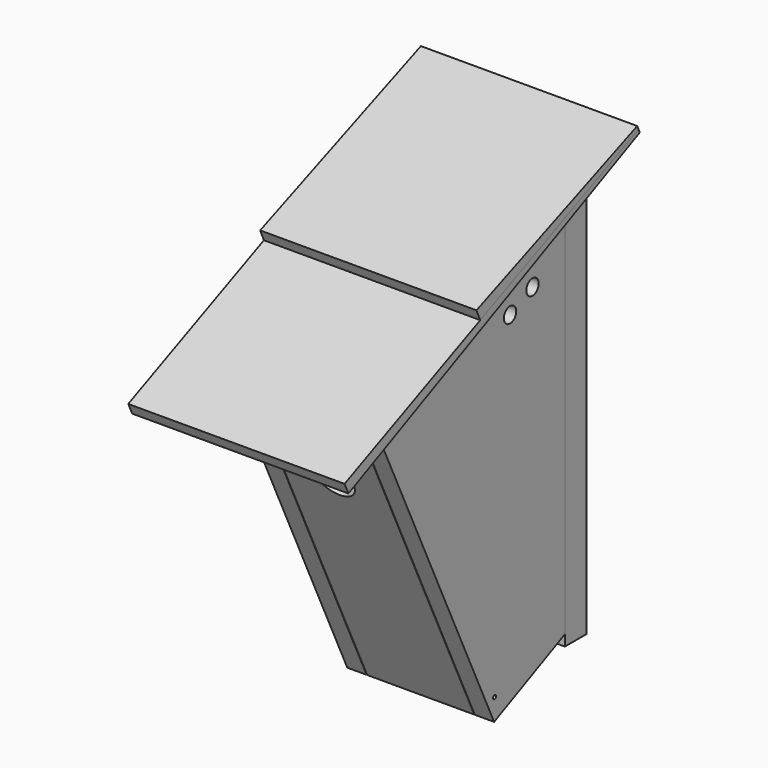
from build123d import *

# Parameters (mm, degrees)
F1_DEPTH       = 355.6
F3_DEPTH       = 60.326
F3_DEPTH_BACK  = 60.326
F5_DEPTH       = 44.45
F7_DEPTH       = 44.45
F8_R           = 1.5875
F8_R_2         = 6.35
F9_DEPTH       = 15.875
F10_R          = 1.5875
F10_R_2        = 6.35
F11_DEPTH      = 15.875
F13_DEPTH      = 15.875
F14_R          = 1.5875
F15_DEPTH      = 25.4
F16_R          = 1.5875
F17_DEPTH      = 25.4
F19_DEPTH      = 88.9
F21_DEPTH      = 88.9
F21_DEPTH_BACK = 88.9
F23_DEPTH      = 60.325
F24_R          = 1.3462
F25_DEPTH      = 38.1
F26_R          = 2.6924
F27_DEPTH      = 0.762
F29_R          = 1.5875
F31_R          = 0.762


with BuildPart() as f1:
    # F0 (on Top) → F1 (new body)
    with BuildSketch(Plane.XY):
        Polygon((60.325, 0), (-60.325, 0), (-60.325, -22.225), (-44.45, -22.225), (-44.45, -38.1), (44.45, -38.1), (44.45, -22.225), (60.325, -22.225), align=None)
    extrude(amount=-F1_DEPTH)

    # F2 (on Right) → F3 (cut, two sides)
    with BuildSketch(Plane.YZ) as f3_sk:
        Polygon((-38.1, -17.7663217757), (0, 0), (-38.1, 0), align=None)
    extrude(amount=-F3_DEPTH, mode=Mode.SUBTRACT)
    extrude(f3_sk.sketch, amount=F3_DEPTH_BACK, mode=Mode.SUBTRACT)


with BuildPart() as f5:
    # F4 (on Right) → F5 (new body, symmetric)
    with BuildSketch(Plane.YZ):
        Polygon((-38.1, -59.8050204882), (-38.1, -17.7663217757), (-209.3013597097, -97.5988268949), (-193.1996039373, -132.129153581), align=None)
    extrude(amount=F5_DEPTH, both=True)


with BuildPart() as f7:
    # F6 (on Right) → F7 (new body, symmetric)
    with BuildSketch(Plane.YZ):
        Polygon((-38.1, -326.5050204882), (-38.1, -284.4663217757), (-107.1493332197, -316.6645546466), (-91.0475774474, -351.1948813327), align=None)
    extrude(amount=F7_DEPTH, both=True)


with BuildPart() as f9:
    # F8 (on face) → F9 (new body, through all)
    with BuildSketch(Plane(origin=(-44.45, 0, 0), x_dir=(0, -1, 0), z_dir=(-1, 0, 0))):
        Polygon((223.6889958289, -104.3078918), (22.225, -10.3636877025), (22.225, -346.6732774023), (94.8749496503, -380.5505052888), align=None)
        with Locations((94.3901964958, -362.808336717)):
            Circle(F8_R, mode=Mode.SUBTRACT)
        with Locations((55.4660997165, -81.9158653491)):
            Circle(F8_R_2, mode=Mode.SUBTRACT)
        with Locations((78.4863175073, -92.6503691973)):
            Circle(F8_R_2, mode=Mode.SUBTRACT)
    extrude(amount=F9_DEPTH)


with BuildPart() as f11:
    # F10 (on face) → F11 (new body, through all)
    with BuildSketch(Plane.YZ.offset(44.45)):
        Polygon((-22.225, -346.6732774023), (-22.225, -10.3636877025), (-223.6889958289, -104.3078918), (-94.8749496503, -380.5505052888), align=None)
        with Locations((-94.3901964958, -362.808336717)):
            Circle(F10_R, mode=Mode.SUBTRACT)
        with Locations((-78.4863175073, -92.6503691973)):
            Circle(F10_R_2, mode=Mode.SUBTRACT)
        with Locations((-55.4660997165, -81.9158653491)):
            Circle(F10_R_2, mode=Mode.SUBTRACT)
    extrude(amount=F11_DEPTH)


with BuildPart() as f13:
    # F12 (on face) → F13 (new body)
    with BuildSketch(Plane(origin=(0, -223.6889958289, -104.3078918), x_dir=(1, 0, 0), z_dir=(0, -0.906307787, -0.4226182617))):
        with BuildLine():
            Line((-2.38125, -6.35), (-44.0436, -6.35))
            Line((-44.0436, -6.35), (-44.0436, -304.8))
            Line((-44.0436, -304.8), (44.0436, -304.8))
            Line((44.0436, -304.8), (44.0436, -6.35))
            Line((44.0436, -6.35), (2.38125, -6.35))
            Line((2.38125, -6.35), (2.38125, -12.7))
            ThreePointArc((2.38125, -12.7), (0, -15.08125), (-2.38125, -12.7))
            Line((-2.38125, -12.7), (-2.38125, -6.35))
        make_face()
        with BuildLine():
            ThreePointArc((17.4625, -90.4875), (0, -107.95), (-17.4625, -90.4875))
            Line((-17.4625, -90.4875), (-17.4625, -68.2625))
            ThreePointArc((-17.4625, -68.2625), (0, -50.8), (17.4625, -68.2625))
            Line((17.4625, -68.2625), (17.4625, -90.4875))
        make_face(mode=Mode.SUBTRACT)
    extrude(amount=-F13_DEPTH)

    # F14 (on face) → F15 (cut)
    with BuildSketch(Plane(origin=(-44.0436, 0, 0), x_dir=(0, -1, 0), z_dir=(-1, 0, 0))):
        with Locations((94.3901964958, -362.808336717)):
            Circle(F14_R)
    extrude(amount=-F15_DEPTH, mode=Mode.SUBTRACT)

    # F16 (on face) → F17 (cut)
    with BuildSketch(Plane.YZ.offset(44.0436)):
        with Locations((-94.3901964958, -362.808336717)):
            Circle(F16_R)
    extrude(amount=-F17_DEPTH, mode=Mode.SUBTRACT)


with BuildPart() as f19:
    # F18 (on Right) → F19 (new body, symmetric)
    with BuildSketch(Plane.YZ):
        Polygon((-284.2382702226, -122.0328074674), (-280.2128312795, -130.6653891389), (19.05, 8.8831608879), (17.708187019, 11.7606881117), align=None)
    extrude(amount=F19_DEPTH, both=True)


with BuildPart() as f21:
    # F20 (on Right) → F21 (new body, two sides)
    with BuildSketch(Plane.YZ) as f21_sk:
        Polygon((-144.8483111348, -60.2686455516), (17.708187019, 11.7606881117), (16.4219489178, 14.6634827216), (-148.7070254382, -51.5602617219), align=None)
    extrude(amount=F21_DEPTH)
    extrude(f21_sk.sketch, amount=-F21_DEPTH_BACK)


with BuildPart() as f23:
    # F22 (on Right) → F23 (new body, symmetric)
    with BuildSketch(Plane.YZ):
        Polygon((19.05, 8.8831608879), (0, 0), (0, -16.5168391121), (19.05, -16.5168391121), align=None)
    extrude(amount=F23_DEPTH, both=True)


with BuildPart() as f25:
    # F24 (on face) → F25 (new body)
    with BuildSketch(Plane(origin=(-60.325, 0, 0), x_dir=(0, -1, 0), z_dir=(-1, 0, 0))):
        with Locations((94.3901964958, -362.808336717)):
            Circle(F24_R)
    extrude(amount=-F25_DEPTH)

    # F26 (on face) → F27 (join)
    with BuildSketch(Plane(origin=(-60.325, 0, 0), x_dir=(0, -1, 0), z_dir=(-1, 0, 0))):
        with Locations((94.3901964958, -362.808336717)):
            Circle(F26_R)
    extrude(amount=F27_DEPTH)


with BuildPart() as f30:
    # F30: sweep along a path in F28
    with BuildLine(Plane.YZ) as f30_path:
        Line((-204.6050142761, -107.6701721783), (-216.1151231714, -113.0374241024))
        ThreePointArc((-216.1151231714, -113.0374241024), (-218.5776898064, -115.7248440056), (-218.4186945357, -119.3664344097))
        Line((-218.4186945357, -119.3664344097), (-216.4059750641, -123.6827252455))
    # F29 (on face) → F30 (sweep)
    with BuildSketch(Plane(origin=(0, -209.3013597097, -97.5988268949), x_dir=(1, 0, 0), z_dir=(0, -0.906307787, -0.4226182617))):
        with Locations((0, -11.1125)):
            Circle(F29_R)
    sweep(path=f30_path.line)

    # F31
    f31_edges = [f30.edges().sort_by_distance(p)[0] for p in [
        (-1.5875, -216.405975, -123.682725),
    ]]
    fillet(f31_edges, radius=F31_R)


solid = Compound([f1.part, f5.part, f7.part, f9.part, f11.part, f13.part, f19.part, f21.part, f23.part, f25.part, f30.part])
